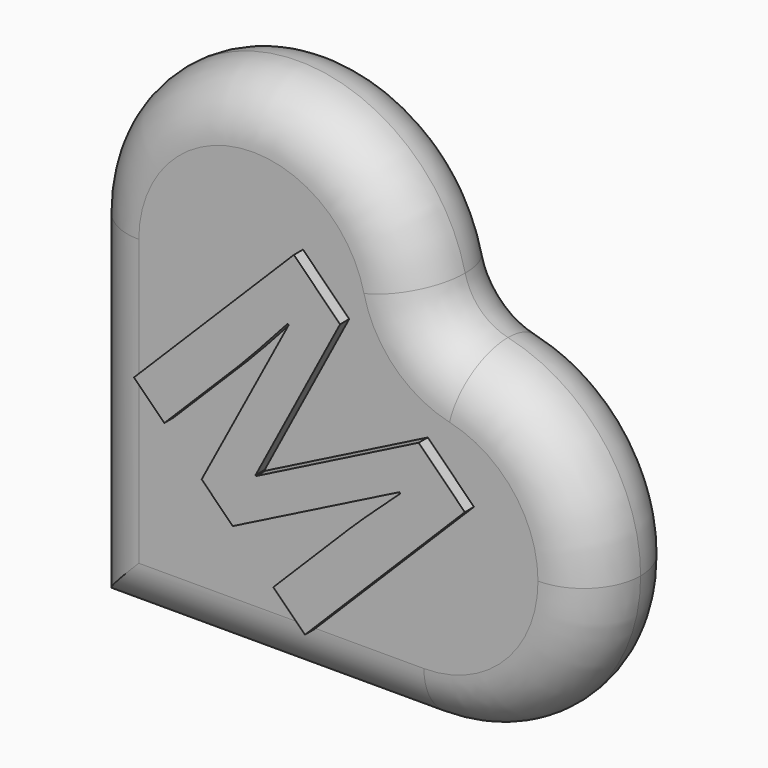
from build123d import *

# Parameters (mm, degrees)
F1_DEPTH     = 6.35
F2_R         = 6.3499
F3_TEXT_SIZE = 35.2777777778
F4_DEPTH     = 7.62


# Not quite as in the source:
# - a fillet or chamfer is up to 0.001 mm smaller than in the source, because OpenCascade refuses the exact size
# - Text() gives the source's letters only with a copy of the font that has no kerning and outlines rounded to 1/6400 em; it was checked with that copy


with BuildPart() as f1:
    # F0 (on Front) → F1 (new body, symmetric)
    with BuildSketch(Plane.XZ):
        with BuildLine():
            ThreePointArc((0, 0), (5.5796158184, -13.4703841816), (19.05, -19.05))
            Line((19.05, -19.05), (19.05, 19.05))
            ThreePointArc((19.05, 19.05), (13.4703841816, 5.5796158184), (0, 0))
        make_face()
        with BuildLine():
            Line((19.05, 19.05), (19.05, -19.05))
            ThreePointArc((19.05, -19.05), (32.5203841816, -13.4703841816), (38.1, 0))
            ThreePointArc((38.1, 0), (32.5203841816, 13.4703841816), (19.05, 19.05))
        make_face()
        with BuildLine():
            Line((-19.05, -19.05), (19.05, -19.05))
            ThreePointArc((19.05, -19.05), (5.5796158184, -13.4703841816), (0, 0))
            ThreePointArc((0, 0), (-13.4703841816, 5.5796158184), (-19.05, 19.05))
            Line((-19.05, 19.05), (-19.05, -19.05))
        make_face()
        with BuildLine():
            ThreePointArc((0, 0), (5.5796158184, 13.4703841816), (19.05, 19.05))
            Line((19.05, 19.05), (-19.05, 19.05))
            ThreePointArc((-19.05, 19.05), (-13.4703841816, 5.5796158184), (0, 0))
        make_face()
        with BuildLine():
            Line((-19.05, 19.05), (19.05, 19.05))
            ThreePointArc((19.05, 19.05), (0, 38.1), (-19.05, 19.05))
        make_face()
        with BuildLine():
            ThreePointArc((0, 0), (13.4703841816, 5.5796158184), (19.05, 19.05))
            ThreePointArc((19.05, 19.05), (5.5796158184, 13.4703841816), (0, 0))
        make_face()
    extrude(amount=F1_DEPTH, both=True)

    # F2 (radius 6.35 in the source; OpenCascade refuses exactly that, so slightly less here)
    f2_edges = [f1.edges().sort_by_distance(p)[0] for p in [
        (38.1, 6.35, 0),
        (19.05, 0, 19.05),
        (38.1, -6.35, 0),
        (19.05, 0, -19.05),
        (0, 6.35, -19.05),
        (0, -6.35, -19.05),
        (-19.05, 6.35, 0),
        (-19.05, -6.35, 0),
        (0, -6.35, 38.1),
        (0, 6.35, 38.1),
    ]]
    fillet(f2_edges, radius=F2_R)

    # F3 (on Front) → F4 (join, symmetric)
    with BuildSketch(Plane.XZ):
        with Locations(Location((-14.4669411352, 8.428482723), (0, 0, -45))):
            Text('M', F3_TEXT_SIZE, font='Open Sans', font_style=FontStyle.BOLD, text_align=(TextAlign.LEFT, TextAlign.BOTTOM))
    extrude(amount=F4_DEPTH, both=True)


solid = f1.part
